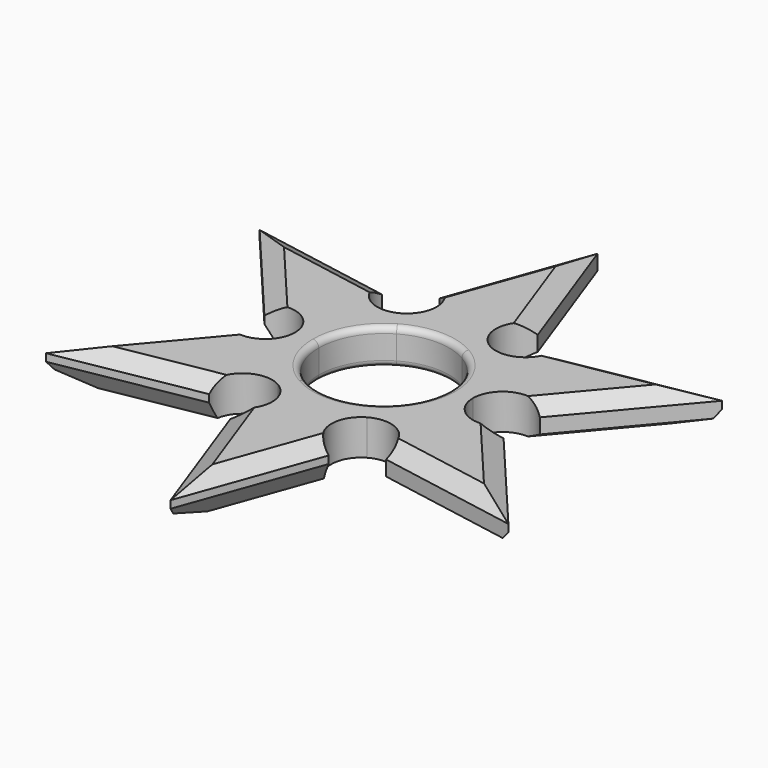
from build123d import *

# Parameters (mm, degrees)
F1_DEPTH     = 6
F2_C1_SIZE2  = 3
F2_C1_SIZE   = 1.7320508076
F2_C2_SIZE2  = 3
F2_C2_SIZE   = 1.7320508076
F2_C3_SIZE2  = 1.7320508076
F2_C3_SIZE   = 3
F2_C4_SIZE2  = 3
F2_C4_SIZE   = 1.7320508076
F2_C5_SIZE2  = 1.7320508076
F2_C5_SIZE   = 3
F2_C6_SIZE2  = 3
F2_C6_SIZE   = 1.7320508076
F2_C7_SIZE2  = 1.7320508076
F2_C7_SIZE   = 3
F2_C8_SIZE2  = 3
F2_C8_SIZE   = 1.7320508076
F2_C9_SIZE2  = 1.7320508076
F2_C9_SIZE   = 3
F2_C10_SIZE2 = 3
F2_C10_SIZE  = 1.7320508076
F2_C11_SIZE2 = 3
F2_C11_SIZE  = 1.7320508076
F2_C12_SIZE2 = 3
F2_C12_SIZE  = 1.7320508076
F2_C13_SIZE2 = 1.7320508076
F2_C13_SIZE  = 3
F2_C14_SIZE2 = 3
F2_C14_SIZE  = 1.7320508076
F2_C15_SIZE2 = 3
F2_C15_SIZE  = 1.7320508076
F2_C16_SIZE2 = 3
F2_C16_SIZE  = 1.7320508076
F2_C17_SIZE2 = 1.7320508076
F2_C17_SIZE  = 3
F2_C18_SIZE2 = 3
F2_C18_SIZE  = 1.7320508076
F2_C19_SIZE2 = 3
F2_C19_SIZE  = 1.7320508076
F2_C20_SIZE2 = 3
F2_C20_SIZE  = 1.7320508076
F2_C21_SIZE2 = 1.7320508076
F2_C21_SIZE  = 3
F2_C22_SIZE2 = 3
F2_C22_SIZE  = 1.7320508076
F2_C23_SIZE2 = 3
F2_C23_SIZE  = 1.7320508076
F2_C24_SIZE2 = 3
F2_C24_SIZE  = 1.7320508076
F3_R         = 1


with BuildPart() as f1:
    # F0 (on Top) → F1 (new body)
    with BuildSketch(Plane.XY):
        with BuildLine():
            ThreePointArc((5.4975, 9.5219493146), (9.5219493146, 5.4975), (10.995, 0))
            Line((10.995, 0), (14.995, 0))
            ThreePointArc((14.995, 0), (17.8875950663, 4.5341861944), (23.2185377782, 3.8221465425))
            Line((23.2185377782, 3.8221465425), (38.9711431703, 22.5))
            Line((38.9711431703, 22.5), (14.9193448919, 18.1967702834))
            ThreePointArc((14.9193448919, 18.1967702834), (12.870517963, 13.2240186428), (7.4975, 12.9860509297))
            Line((7.4975, 12.9860509297), (5.4975, 9.5219493146))
        make_face()
        with BuildLine():
            ThreePointArc((-5.4975, 9.5219493146), (0, 10.995), (5.4975, 9.5219493146))
            Line((5.4975, 9.5219493146), (7.4975, 12.9860509297))
            ThreePointArc((7.4975, 12.9860509297), (5.0170771033, 17.7582048372), (8.2991928863, 22.0189168259))
            Line((8.2991928863, 22.0189168259), (0, 45))
            Line((0, 45), (-8.2991928863, 22.0189168259))
            ThreePointArc((-8.2991928863, 22.0189168259), (-5.0170771033, 17.7582048372), (-7.4975, 12.9860509297))
            Line((-7.4975, 12.9860509297), (-5.4975, 9.5219493146))
        make_face()
        with BuildLine():
            ThreePointArc((-10.995, 0), (-9.5219493146, 5.4975), (-5.4975, 9.5219493146))
            Line((-5.4975, 9.5219493146), (-7.4975, 12.9860509297))
            ThreePointArc((-7.4975, 12.9860509297), (-12.870517963, 13.2240186428), (-14.9193448919, 18.1967702834))
            Line((-14.9193448919, 18.1967702834), (-38.9711431703, 22.5))
            Line((-38.9711431703, 22.5), (-23.2185377782, 3.8221465425))
            ThreePointArc((-23.2185377782, 3.8221465425), (-17.8875950663, 4.5341861944), (-14.995, 0))
            Line((-14.995, 0), (-10.995, 0))
        make_face()
        with BuildLine():
            Line((-7.4975, -12.9860509297), (-5.4975, -9.5219493146))
            ThreePointArc((-5.4975, -9.5219493146), (-9.5219493146, -5.4975), (-10.995, 0))
            Line((-10.995, 0), (-14.995, 0))
            ThreePointArc((-14.995, 0), (-17.8875950663, -4.5341861944), (-23.2185377782, -3.8221465425))
            Line((-23.2185377782, -3.8221465425), (-38.9711431703, -22.5))
            Line((-38.9711431703, -22.5), (-14.9193448919, -18.1967702834))
            ThreePointArc((-14.9193448919, -18.1967702834), (-12.870517963, -13.2240186428), (-7.4975, -12.9860509297))
        make_face()
        with BuildLine():
            Line((7.4975, -12.9860509297), (5.4975, -9.5219493146))
            ThreePointArc((5.4975, -9.5219493146), (0, -10.995), (-5.4975, -9.5219493146))
            Line((-5.4975, -9.5219493146), (-7.4975, -12.9860509297))
            ThreePointArc((-7.4975, -12.9860509297), (-5.0170771033, -17.7582048372), (-8.2991928863, -22.0189168259))
            Line((-8.2991928863, -22.0189168259), (0, -45))
            Line((0, -45), (8.2991928863, -22.0189168259))
            ThreePointArc((8.2991928863, -22.0189168259), (5.0170771033, -17.7582048372), (7.4975, -12.9860509297))
        make_face()
        with BuildLine():
            Line((14.995, 0), (10.995, 0))
            ThreePointArc((10.995, 0), (9.5219493146, -5.4975), (5.4975, -9.5219493146))
            Line((5.4975, -9.5219493146), (7.4975, -12.9860509297))
            ThreePointArc((7.4975, -12.9860509297), (12.870517963, -13.2240186428), (14.9193448919, -18.1967702834))
            Line((14.9193448919, -18.1967702834), (38.9711431703, -22.5))
            Line((38.9711431703, -22.5), (23.2185377782, -3.8221465425))
            ThreePointArc((23.2185377782, -3.8221465425), (17.8875950663, -4.5341861944), (14.995, 0))
        make_face()
    extrude(amount=F1_DEPTH)

    # F2: chamfer of 3 x 1.7320508076 on 24 edges, made by hand

    # F2_c1
    f2_c1_edges = [f1.edges().sort_by_distance(p)[0] for p in [
        (31.0948404742, 13.1610732713, 0),
    ]]
    f2_c1_side = f1.faces().sort_by_distance((31.0948404742, 13.1610732713, 0.0346410162))[0]
    chamfer(f2_c1_edges, length=F2_C1_SIZE, length2=F2_C1_SIZE2, reference=f2_c1_side)

    # F2_c2
    f2_c2_edges = [f1.edges().sort_by_distance(p)[0] for p in [
        (31.0948404742, 13.1610732713, 6),
    ]]
    f2_c2_side = f1.faces().sort_by_distance((31.0948404742, 13.1610732713, 5.9653589838))[0]
    chamfer(f2_c2_edges, length=F2_C2_SIZE, length2=F2_C2_SIZE2, reference=f2_c2_side)

    # F2_c3
    f2_c3_edges = [f1.edges().sort_by_distance(p)[0] for p in [
        (24.6342857936, 19.9349198346, 0),
    ]]
    f2_c3_side = f1.faces().sort_by_distance((24.6342857936, 19.9349198346, 0.0346410162))[0]
    chamfer(f2_c3_edges, length=F2_C3_SIZE, length2=F2_C3_SIZE2, reference=f2_c3_side)

    # F2_c4
    f2_c4_edges = [f1.edges().sort_by_distance(p)[0] for p in [
        (24.6342857936, 19.9349198346, 6),
    ]]
    f2_c4_side = f1.faces().sort_by_distance((24.6342857936, 19.9349198346, 5.9653589838))[0]
    chamfer(f2_c4_edges, length=F2_C4_SIZE, length2=F2_C4_SIZE2, reference=f2_c4_side)

    # F2_c5
    f2_c5_edges = [f1.edges().sort_by_distance(p)[0] for p in [
        (4.1495964431, 33.509458413, 0),
    ]]
    f2_c5_side = f1.faces().sort_by_distance((4.1170149125, 33.4976921961, 0))[0]
    chamfer(f2_c5_edges, length=F2_C5_SIZE, length2=F2_C5_SIZE2, reference=f2_c5_side)

    # F2_c6
    f2_c6_edges = [f1.edges().sort_by_distance(p)[0] for p in [
        (4.1495964431, 33.509458413, 6),
    ]]
    f2_c6_side = f1.faces().sort_by_distance((4.1495964431, 33.509458413, 5.9653589838))[0]
    chamfer(f2_c6_edges, length=F2_C6_SIZE, length2=F2_C6_SIZE2, reference=f2_c6_side)

    # F2_c7
    f2_c7_edges = [f1.edges().sort_by_distance(p)[0] for p in [
        (-4.9470041023, 31.3013772186, 0),
    ]]
    f2_c7_side = f1.faces().sort_by_distance((-4.9144225717, 31.2896110018, 0))[0]
    chamfer(f2_c7_edges, length=F2_C7_SIZE, length2=F2_C7_SIZE2, reference=f2_c7_side)

    # F2_c8
    f2_c8_edges = [f1.edges().sort_by_distance(p)[0] for p in [
        (-4.9470041023, 31.3013772186, 6),
    ]]
    f2_c8_side = f1.faces().sort_by_distance((-4.9470041023, 31.3013772186, 5.9653589838))[0]
    chamfer(f2_c8_edges, length=F2_C8_SIZE, length2=F2_C8_SIZE2, reference=f2_c8_side)

    # F2_c9
    f2_c9_edges = [f1.edges().sort_by_distance(p)[0] for p in [
        (-26.9452440311, 20.3483851417, 0),
    ]]
    f2_c9_side = f1.faces().sort_by_distance((-26.9513449538, 20.3142856, 0))[0]
    chamfer(f2_c9_edges, length=F2_C9_SIZE, length2=F2_C9_SIZE2, reference=f2_c9_side)

    # F2_c10
    f2_c10_edges = [f1.edges().sort_by_distance(p)[0] for p in [
        (-26.9452440311, 20.3483851417, 6),
    ]]
    f2_c10_side = f1.faces().sort_by_distance((-26.9452440311, 20.3483851417, 5.9653589838))[0]
    chamfer(f2_c10_edges, length=F2_C10_SIZE, length2=F2_C10_SIZE2, reference=f2_c10_side)

    # F2_c11
    f2_c11_edges = [f1.edges().sort_by_distance(p)[0] for p in [
        (-29.581289896, 11.3664573841, 0),
    ]]
    f2_c11_side = f1.faces().sort_by_distance((-29.5548092879, 11.3887907089, 0))[0]
    chamfer(f2_c11_edges, length=F2_C11_SIZE, length2=F2_C11_SIZE2, reference=f2_c11_side)

    # F2_c12
    f2_c12_edges = [f1.edges().sort_by_distance(p)[0] for p in [
        (-29.581289896, 11.3664573841, 6),
    ]]
    f2_c12_side = f1.faces().sort_by_distance((-29.581289896, 11.3664573841, 5.9653589838))[0]
    chamfer(f2_c12_edges, length=F2_C12_SIZE, length2=F2_C12_SIZE2, reference=f2_c12_side)

    # F2_c13
    f2_c13_edges = [f1.edges().sort_by_distance(p)[0] for p in [
        (-31.0948404742, -13.1610732713, 0),
    ]]
    f2_c13_side = f1.faces().sort_by_distance((-31.0683598662, -13.1834065961, 0))[0]
    chamfer(f2_c13_edges, length=F2_C13_SIZE, length2=F2_C13_SIZE2, reference=f2_c13_side)

    # F2_c14
    f2_c14_edges = [f1.edges().sort_by_distance(p)[0] for p in [
        (-31.0948404742, -13.1610732713, 6),
    ]]
    f2_c14_side = f1.faces().sort_by_distance((-31.0948404742, -13.1610732713, 5.9653589838))[0]
    chamfer(f2_c14_edges, length=F2_C14_SIZE, length2=F2_C14_SIZE2, reference=f2_c14_side)

    # F2_c15
    f2_c15_edges = [f1.edges().sort_by_distance(p)[0] for p in [
        (-24.6342857936, -19.9349198346, 0),
    ]]
    f2_c15_side = f1.faces().sort_by_distance((-24.6403867163, -19.9008202929, 0))[0]
    chamfer(f2_c15_edges, length=F2_C15_SIZE, length2=F2_C15_SIZE2, reference=f2_c15_side)

    # F2_c16
    f2_c16_edges = [f1.edges().sort_by_distance(p)[0] for p in [
        (-24.6342857936, -19.9349198346, 6),
    ]]
    f2_c16_side = f1.faces().sort_by_distance((-24.6342857936, -19.9349198346, 5.9653589838))[0]
    chamfer(f2_c16_edges, length=F2_C16_SIZE, length2=F2_C16_SIZE2, reference=f2_c16_side)

    # F2_c17
    f2_c17_edges = [f1.edges().sort_by_distance(p)[0] for p in [
        (-4.1495964431, -33.509458413, 0),
    ]]
    f2_c17_side = f1.faces().sort_by_distance((-4.1170149125, -33.4976921961, 0))[0]
    chamfer(f2_c17_edges, length=F2_C17_SIZE, length2=F2_C17_SIZE2, reference=f2_c17_side)

    # F2_c18
    f2_c18_edges = [f1.edges().sort_by_distance(p)[0] for p in [
        (-4.1495964431, -33.509458413, 6),
    ]]
    f2_c18_side = f1.faces().sort_by_distance((-4.1495964431, -33.509458413, 5.9653589838))[0]
    chamfer(f2_c18_edges, length=F2_C18_SIZE, length2=F2_C18_SIZE2, reference=f2_c18_side)

    # F2_c19
    f2_c19_edges = [f1.edges().sort_by_distance(p)[0] for p in [
        (4.9470041023, -31.3013772186, 0),
    ]]
    f2_c19_side = f1.faces().sort_by_distance((4.9144225717, -31.2896110018, 0))[0]
    chamfer(f2_c19_edges, length=F2_C19_SIZE, length2=F2_C19_SIZE2, reference=f2_c19_side)

    # F2_c20
    f2_c20_edges = [f1.edges().sort_by_distance(p)[0] for p in [
        (4.9470041023, -31.3013772186, 6),
    ]]
    f2_c20_side = f1.faces().sort_by_distance((4.9470041023, -31.3013772186, 5.9653589838))[0]
    chamfer(f2_c20_edges, length=F2_C20_SIZE, length2=F2_C20_SIZE2, reference=f2_c20_side)

    # F2_c21
    f2_c21_edges = [f1.edges().sort_by_distance(p)[0] for p in [
        (26.9452440311, -20.3483851417, 0),
    ]]
    f2_c21_side = f1.faces().sort_by_distance((26.9513449538, -20.3142856, 0))[0]
    chamfer(f2_c21_edges, length=F2_C21_SIZE, length2=F2_C21_SIZE2, reference=f2_c21_side)

    # F2_c22
    f2_c22_edges = [f1.edges().sort_by_distance(p)[0] for p in [
        (26.9452440311, -20.3483851417, 6),
    ]]
    f2_c22_side = f1.faces().sort_by_distance((26.9452440311, -20.3483851417, 5.9653589838))[0]
    chamfer(f2_c22_edges, length=F2_C22_SIZE, length2=F2_C22_SIZE2, reference=f2_c22_side)

    # F2_c23
    f2_c23_edges = [f1.edges().sort_by_distance(p)[0] for p in [
        (29.581289896, -11.3664573841, 0),
    ]]
    f2_c23_side = f1.faces().sort_by_distance((29.5548092879, -11.3887907089, 0))[0]
    chamfer(f2_c23_edges, length=F2_C23_SIZE, length2=F2_C23_SIZE2, reference=f2_c23_side)

    # F2_c24
    f2_c24_edges = [f1.edges().sort_by_distance(p)[0] for p in [
        (29.581289896, -11.3664573841, 6),
    ]]
    f2_c24_side = f1.faces().sort_by_distance((29.581289896, -11.3664573841, 5.9653589838))[0]
    chamfer(f2_c24_edges, length=F2_C24_SIZE, length2=F2_C24_SIZE2, reference=f2_c24_side)

    # F3
    f3_edges = [f1.edges().sort_by_distance(p)[0] for p in [
        (-10.995, 0, 0),
        (-10.995, 0, 6),
    ]]
    fillet(f3_edges, radius=F3_R)


solid = f1.part
